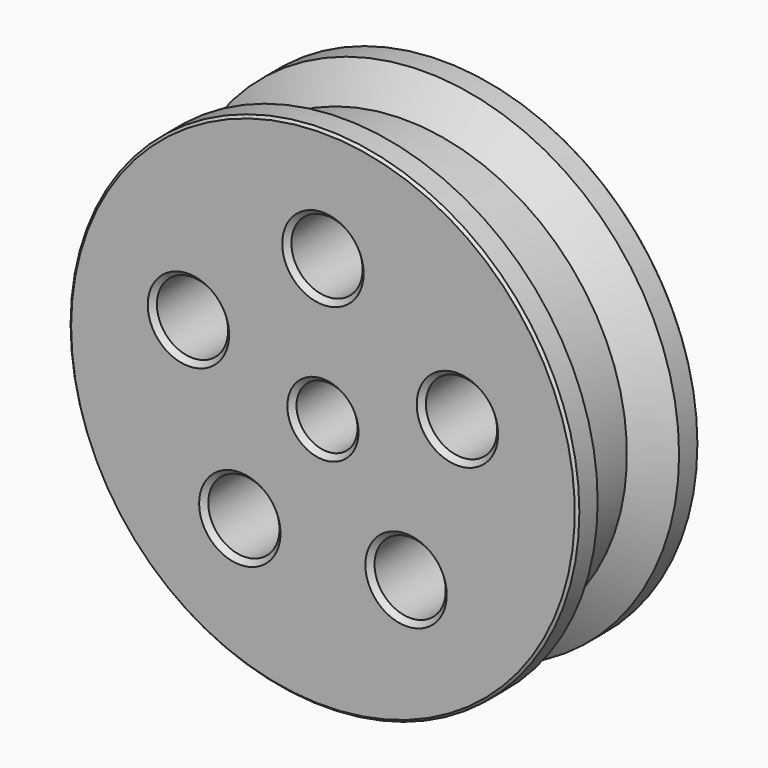
from build123d import *

# Parameters (mm, degrees)
F2_R     = 6
F3_DEPTH = 40.001
F4_R     = 7
F5_DEPTH = 30
F6_SIZE  = 0.5
F7_SIZE  = 0.99999


# Not quite as in the source:
# - a fillet or chamfer is up to 0.001 mm smaller than in the source, because OpenCascade refuses the exact size


with BuildPart() as f1:
    # F0 (on Top) → F1 (revolve)
    with BuildSketch(Plane.XY):
        Polygon((-50, -40), (0, -40), (0, 0), (-10, 0), (-19.7979589711, -10), (-50, -10), (-50, -15), (-43.7550020016, -20), (-43.7550020016, -30), (-50, -35), align=None)
    revolve(axis=Axis((0, -20, 0), (0, -1, 0)))

    # F2 (on face) → F3 (cut, through all)
    with BuildSketch(Plane(origin=(0, 0, 0), x_dir=(-1, 0, 0), z_dir=(0, 1, 0))):
        Circle(F2_R)
    extrude(amount=-F3_DEPTH, mode=Mode.SUBTRACT)

    # F4 (on face) → F5 (cut)
    with BuildSketch(Plane(origin=(0, -10, 0), x_dir=(-1, 0, 0), z_dir=(0, 1, 0))):
        with Locations((0, 27.7979589711)):
            Circle(F4_R)
        with Locations((26.4374300192, 8.590041731)):
            Circle(F4_R)
        with Locations((16.3392303271, -22.4890212166)):
            Circle(F4_R)
        with Locations((-16.3392303271, -22.4890212166)):
            Circle(F4_R)
        with Locations((-26.4374300192, 8.590041731)):
            Circle(F4_R)
    extrude(amount=-F5_DEPTH, mode=Mode.SUBTRACT)

    # F6
    f6_edges = [f1.edges().sort_by_distance(p)[0] for p in [
        (50, -40, 0),
        (50, -10, 0),
    ]]
    chamfer(f6_edges, length=F6_SIZE)

    # F7 (size 1 in the source; OpenCascade refuses exactly that, so slightly less here)
    f7_edges = [f1.edges().sort_by_distance(p)[0] for p in [
        (7, -10, 27.797959),
        (-19.43743, -10, 8.590042),
        (-9.33923, -10, -22.489021),
        (23.33923, -10, -22.489021),
        (33.43743, -10, 8.590042),
        (-9.33923, -40, -22.489021),
        (-19.43743, -40, 8.590042),
        (33.43743, -40, 8.590042),
        (23.33923, -40, -22.489021),
        (6, -40, 0),
        (7, -40, 27.797959),
    ]]
    chamfer(f7_edges, length=F7_SIZE)


solid = f1.part
